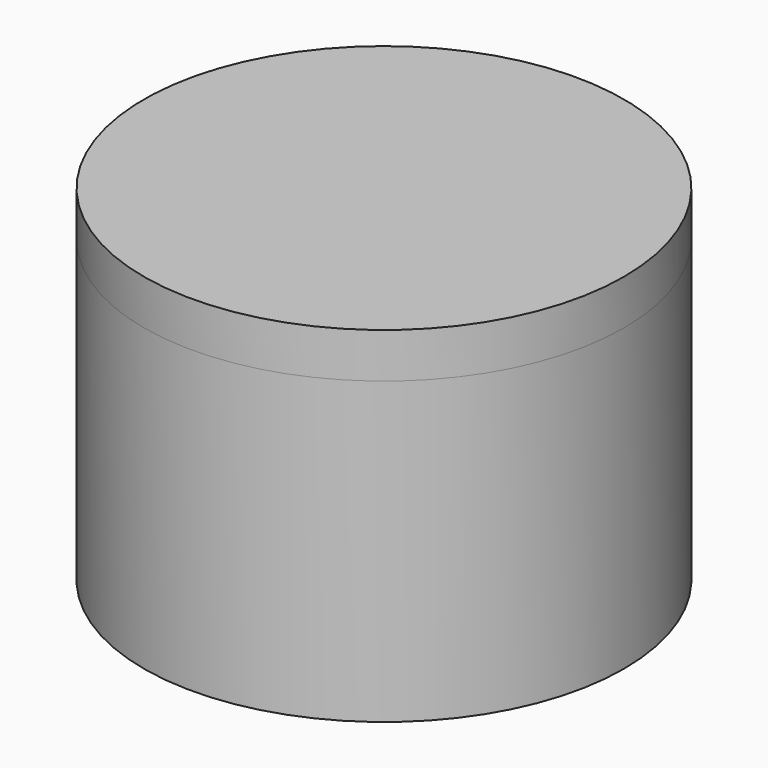
from build123d import *

# Parameters (mm, degrees)
F0_R     = 12.7
F1_DEPTH = 15.875
F2_R     = 12.7
F3_DEPTH = 2.38125


# Not quite as in the source:
# - a length typed as a fraction of an inch, garbled in the dataset ("3 / 203.2 mm" for 3/8 in), is restored


with BuildPart() as f1:
    # F0 (on Top) → F1 (new body)
    with BuildSketch(Plane.XY):
        Circle(F0_R)
    extrude(amount=F1_DEPTH)


with BuildPart() as f3:
    # F2 (on face) → F3 (new body)
    with BuildSketch(Plane.XY.offset(15.875)):
        Circle(F2_R)
    extrude(amount=F3_DEPTH)


solid = Compound([f1.part, f3.part])
